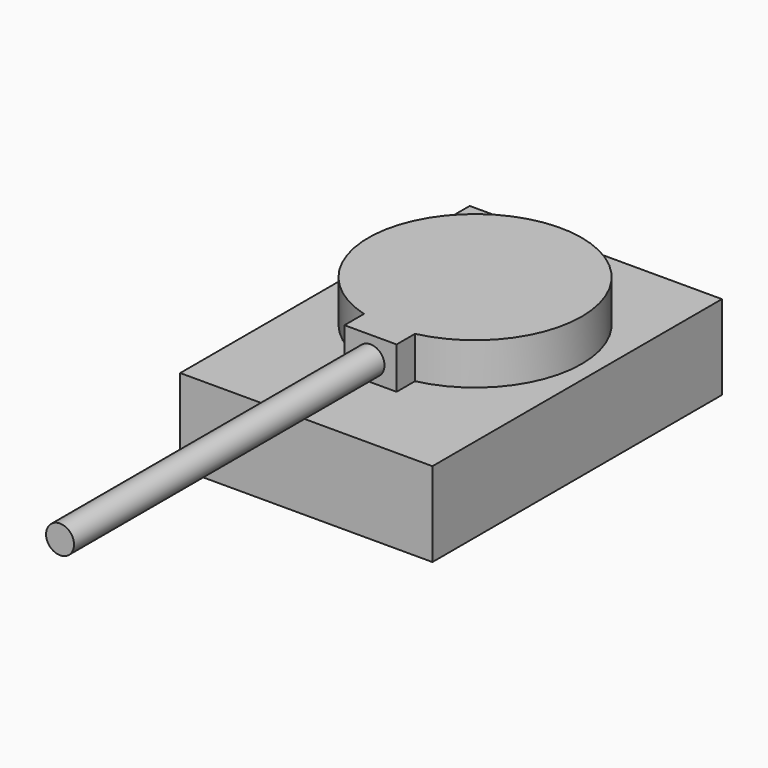
from build123d import *

# Parameters (mm, degrees)
F0_W     = 66.0297609866
F0_H     = 94.7342179716
F1_DEPTH = 22.098
F3_DEPTH = 10.922
F4_R     = 3.6634356374
F5_DEPTH = 101.6
F6_R     = 9.1104151175
F7_DEPTH = 1.778


with BuildPart() as f1:
    # F0 (on Top) → F1 (new body)
    with BuildSketch(Plane.XY):
        with Locations((-0.6452407688, -7.0482958108)):
            Rectangle(F0_W, F0_H)
    extrude(amount=F1_DEPTH)


with BuildPart() as f3:
    # F2 (on face) → F3 (new body)
    with BuildSketch(Plane.XY.offset(22.098)):
        with BuildLine():
            ThreePointArc((6.0832463205, -27.2641839674), (21.797644794, -17.470097156), (27.9345952755, 0))
            ThreePointArc((27.9345952755, 0), (-16.8675799898, 22.2671587432), (-7.5644949102, -26.890891208))
            ThreePointArc((-7.5644949102, -26.890891208), (-0.7637808699, -27.9241517685), (6.0832463205, -27.2641839674))
        make_face()
        with BuildLine():
            ThreePointArc((6.0832463205, -27.2641839674), (-0.7637808699, -27.9241517685), (-7.5644949102, -26.890891208))
            Line((-7.5644949102, -26.890891208), (-7.5644949102, -33.2837412526))
            Line((-7.5644949102, -33.2837412526), (6.0832463205, -33.2837412526))
            Line((6.0832463205, -33.2837412526), (6.0832463205, -27.2641839674))
        make_face()
    extrude(amount=F3_DEPTH)


with BuildPart() as f5:
    # F4 (on face) → F5 (new body)
    with BuildSketch(Plane.XZ.offset(33.2837412526)):
        with Locations((-0.7406242949, 27.171716094)):
            Circle(F4_R)
    extrude(amount=F5_DEPTH)


with BuildPart() as f7:
    # F6 (on face) → F7 (new body)
    with BuildSketch(Plane(origin=(-33.6601212621, 0, 0), x_dir=(0, -1, 0), z_dir=(-1, 0, 0))):
        with Locations((38.9891192317, 10.5448067188)):
            Circle(F6_R)
    extrude(amount=F7_DEPTH)


solid = Compound([f1.part, f3.part, f5.part, f7.part])
